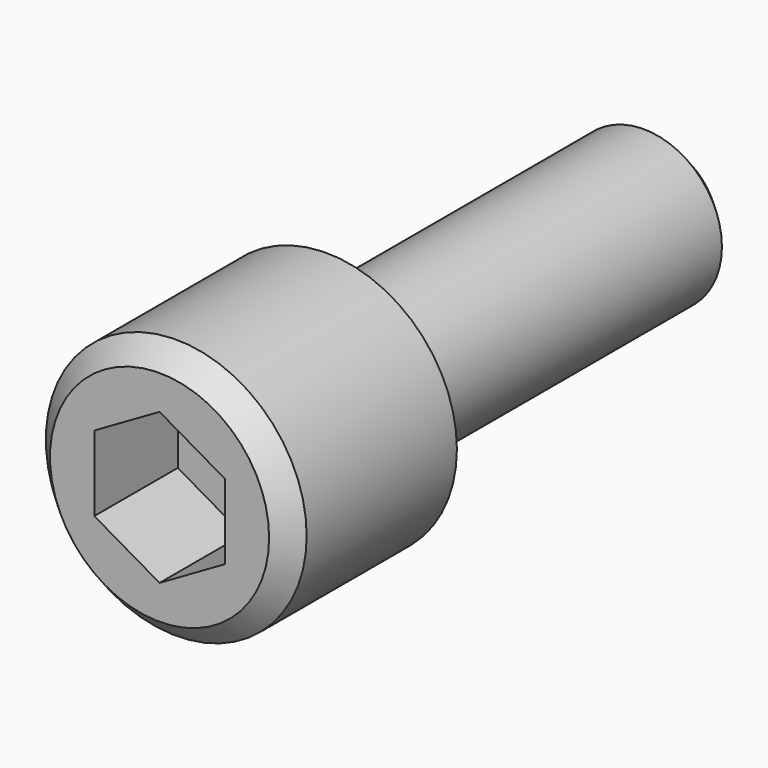
from build123d import *

# Parameters (mm, degrees)
F0_R     = 1.5
F1_DEPTH = 8
F0_R_2   = 2.5
F2_DEPTH = 4
F4_DEPTH = 2
F5_SIZE  = 0.4


# Not quite as in the source:
# - a feature names something its author has since deleted; it is built from what else it names


with BuildPart() as f1:
    # F0 (on Front) → F1 (new body)
    with BuildSketch(Plane.XZ):
        Circle(F0_R)
    extrude(amount=-F1_DEPTH)

    # F0 (on Front) → F2 (join)
    with BuildSketch(Plane.XZ):
        Circle(F0_R_2)
        Circle(F0_R, mode=Mode.SUBTRACT)
        Circle(F0_R)
    extrude(amount=F2_DEPTH)

    # F3 (on face) → F4 (cut)
    with BuildSketch(Plane.XZ.offset(4)):
        Polygon((1.25, -0.7216878365), (1.25, 0.7216878365), (0, 1.443375673), (-1.25, 0.7216878365), (-1.25, -0.7216878365), (0, -1.443375673), align=None)
    extrude(amount=-F4_DEPTH, mode=Mode.SUBTRACT)

    # F5
    f5_edges = [f1.edges().sort_by_distance(p)[0] for p in [
        (-2.5, -4, 0),
        (-1.5, 8, 0),
    ]]
    chamfer(f5_edges, length=F5_SIZE)


solid = f1.part
